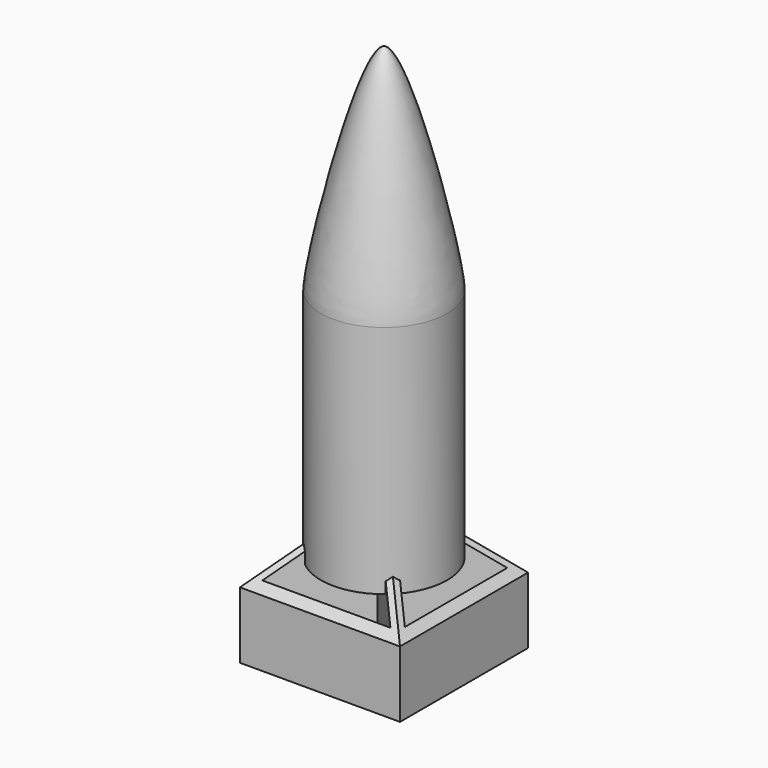
from build123d import *

# Parameters (mm, degrees)
F3_START    = -28.7
F2_W        = 20
F2_H        = 20
F3_DEPTH    = 13.3
F4_T1_DEPTH = 45.7168298797
F4_T3_DEPTH = 45.7168298797


# Not quite as in the source:
# - a fillet or chamfer that OpenCascade refuses, or shapes differently, is made with other operations: its cross-section is extruded or revolved along the edge and cut away or added


with BuildPart() as f1:
    # F0 (on Front) → F1 (revolve)
    with BuildSketch(Plane.XZ):
        with BuildLine():
            Line((2.8410700233, -29.3871536851), (5.784040158, -29.3871536851))
            Line((5.784040158, -29.3871536851), (7.5652169337, -31.1683304608))
            Line((7.5652169337, -31.1683304608), (7.879216224, -31.1683304608))
            Line((7.879216224, -31.1683304608), (7.879216224, -1.8401825801))
            add(Edge.make_bspline(
                [(0, 24.9539222568), (2.5612364989, 24.9539222568), (7.879216224, 1.3124344186), (7.879216224, -1.8401825801)],
                knots=[0, 0, 0, 0, 27.9285893363, 27.9285893363, 27.9285893363, 27.9285893363], degree=3))
            Line((0, 24.9539222568), (0, 0))
            Line((0, 0), (0, -25.4955813289))
            Line((0, -25.4955813289), (1.4129093615, -27.9308501631))
            Line((1.4129093615, -27.9308501631), (1.4129093615, -30.8610778302))
            Line((1.4129093615, -30.8610778302), (3.4415575342, -30.8610778302))
            Line((3.4415575342, -30.8610778302), (2.8410700233, -29.3871536851))
        make_face()
    revolve(axis=Axis((0, 0, 12.4769611284), (0, 0, -1)))


with BuildPart() as f3:
    # F2 (on Top) → F3 (new body)
    with BuildSketch(Plane.XY.offset(F3_START)):
        Rectangle(F2_W, F2_H)
        Polygon((-1, 0), (-8.9999996126, -7.9999996126), (-8.9999996126, 7.9999996126), align=None, mode=Mode.SUBTRACT)
        Polygon((0, -1), (7.9999996126, -8.9999996126), (-7.9999996126, -8.9999996126), align=None, mode=Mode.SUBTRACT)
        Polygon((-7.9999996126, 8.9999996126), (7.9999996126, 8.9999996126), (0, 1), align=None, mode=Mode.SUBTRACT)
        Polygon((8.9999996126, 7.9999996126), (8.9999996126, -7.9999996126), (1, 0), align=None, mode=Mode.SUBTRACT)
    extrude(amount=-F3_DEPTH)

    # F4: chamfer of 5 on 4 edges, made by hand

    # F4_s2 → F4_t1 (cut)
    with BuildSketch(Plane.XZ.offset(-22.8584149398)):
        Polygon((10, -33.7), (5, -28.7), (10, -28.7), align=None)
        Polygon((-10, -33.7), (-5, -28.7), (-10, -28.7), align=None)
    extrude(amount=F4_T1_DEPTH, mode=Mode.SUBTRACT)

    # F4_s4 → F4_t3 (cut)
    with BuildSketch(Plane.YZ.offset(-22.8584149398)):
        Polygon((10, -33.7), (5, -28.7), (10, -28.7), align=None)
        Polygon((-10, -33.7), (-5, -28.7), (-10, -28.7), align=None)
    extrude(amount=F4_T3_DEPTH, mode=Mode.SUBTRACT)


solid = Compound([f1.part, f3.part])
